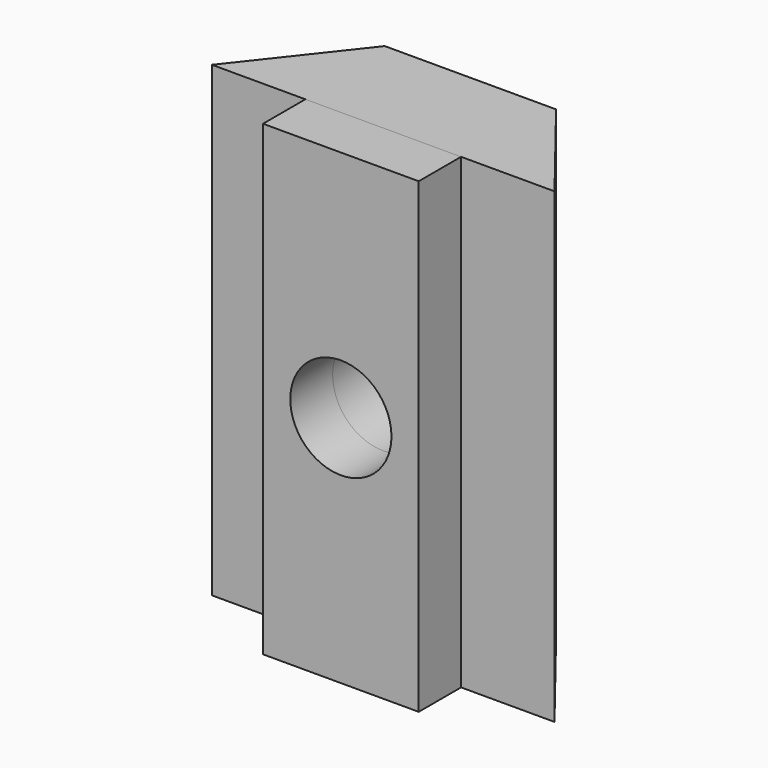
from build123d import *
from build123d import SkipClean  # not in build123d's __all__

# Parameters (mm, degrees)
F1_DEPTH = 15
F2_R     = 1.625
F3_DEPTH = 25
F4_DEPTH = 2
F5_W     = 5
F5_H     = 15
F5_R     = 1.625
F6_DEPTH = 1.7


with BuildPart() as f1:
    # F0 (on Top) → F1 (new body)
    with BuildSketch(Plane.XY):
        Polygon((14.889925763, 7.4500351371), (12.139925763, 7.4500351371), (9.389925763, 7.4500351371), (6.639925763, 3.9500351371), (12.139925763, 3.9500351371), (17.639925763, 3.9500351371), align=None)
    extrude(amount=F1_DEPTH)

    # F2 (on face) → F3 (cut)
    with BuildSketch(Plane(origin=(0, 7.4500351371, 0), x_dir=(-1, 0, 0), z_dir=(0, 1, 0))):
        with Locations((-12.139925763, 7.5)):
            Circle(F2_R)
    extrude(amount=-F3_DEPTH, mode=Mode.SUBTRACT)

    # F2 (on face) → F4 (cut)
    with BuildSketch(Plane(origin=(0, 7.4500351371, 0), x_dir=(-1, 0, 0), z_dir=(0, 1, 0))):
        Polygon((-9.139925763, 5.7679491924), (-9.139925763, 9.2320508076), (-9.389925763, 9.3763883749), (-9.389925763, 5.6236116251), align=None)
        Polygon((-9.389925763, 5.6236116251), (-9.389925763, 9.3763883749), (-12.139925763, 10.9641016151), (-14.889925763, 9.3763883749), (-14.889925763, 5.6236116251), (-12.139925763, 4.0358983849), align=None)
        with Locations((-12.139925763, 7.5)):
            Circle(F2_R, mode=Mode.SUBTRACT)
    extrude(amount=-F4_DEPTH, mode=Mode.SUBTRACT)

    # F5 (on face) → F6 (join)
    with BuildSketch(Plane.XZ.offset(-3.9500351371)):
        with Locations((12.139925763, 7.5)):
            Rectangle(F5_W, F5_H)
        with Locations((12.139925763, 7.5)):
            Circle(F5_R, mode=Mode.SUBTRACT)
    with SkipClean():  # cleaning this boolean's faces spoils the solid; the shape is the same uncleaned
        extrude(amount=F6_DEPTH)


solid = f1.part
